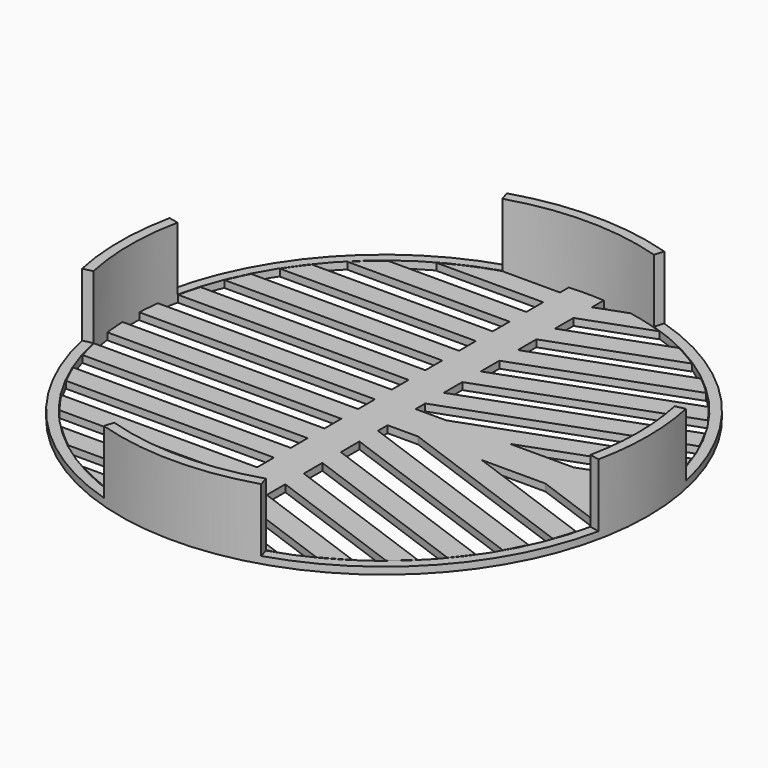
from build123d import *

# Parameters (mm, degrees)
F1_R     = 37.5
F1_R_2   = 36.1
F2_DEPTH = 10
F3_R     = 36
F4_DEPTH = 1
F5_DEPTH = 1
F7_DEPTH = 9


with BuildPart() as f2:
    # F1 (on Top) → F2 (new body)
    with BuildSketch(Plane.XY):
        Circle(F1_R)
        Circle(F1_R_2, mode=Mode.SUBTRACT)
    extrude(amount=F2_DEPTH)

    # F6 (on face) → F7 (cut)
    with BuildSketch(Plane.XY.offset(10)):
        with BuildLine():
            Line((-36.7841187228, 7.7902894544), (-35.316667178, 7.4795066305))
            ThreePointArc((-35.316667178, 7.4795066305), (-26.7003142326, 24.2961564837), (-10.7688596698, 34.4563733061))
            Line((-10.7688596698, 34.4563733061), (-11.2163192129, 35.8880785682))
            ThreePointArc((-11.2163192129, 35.8880785682), (-27.8097455719, 25.3056920716), (-36.7841187228, 7.7902894544))
        make_face()
        with BuildLine():
            Line((35.316667178, 7.4795066305), (36.7841187228, 7.7902894544))
            ThreePointArc((36.7841187228, 7.7902894544), (27.8097455719, 25.3056920716), (11.2163192129, 35.8880785682))
            Line((11.2163192129, 35.8880785682), (10.7688596698, 34.4563733061))
            ThreePointArc((10.7688596698, 34.4563733061), (26.7003142326, 24.2961564837), (35.316667178, 7.4795066305))
        make_face()
        with BuildLine():
            Line((10.7688596698, -34.4563733061), (11.2163192129, -35.8880785682))
            ThreePointArc((11.2163192129, -35.8880785682), (27.8097455719, -25.3056920716), (36.7841187228, -7.7902894544))
            Line((36.7841187228, -7.7902894544), (35.316667178, -7.4795066305))
            ThreePointArc((35.316667178, -7.4795066305), (26.7003142326, -24.2961564837), (10.7688596698, -34.4563733061))
        make_face()
        with BuildLine():
            Line((-35.316667178, -7.4795066305), (-36.7841187228, -7.7902894544))
            ThreePointArc((-36.7841187228, -7.7902894544), (-27.8097455719, -25.3056920716), (-11.2163192129, -35.8880785682))
            Line((-11.2163192129, -35.8880785682), (-10.7688596698, -34.4563733061))
            ThreePointArc((-10.7688596698, -34.4563733061), (-26.7003142326, -24.2961564837), (-35.316667178, -7.4795066305))
        make_face()
    extrude(amount=-F7_DEPTH, mode=Mode.SUBTRACT)


with BuildPart() as f4:
    # F3 (on Top) → F4 (new body)
    with BuildSketch(Plane.XY):
        Circle(F3_R)
    extrude(amount=F4_DEPTH)

    # F0 (on Top) → F5 (cut)
    with BuildSketch(Plane.XY):
        Polygon((-2.4902910933, -34.3626238759), (-11.0826741202, -34.3626238759), (-10.311164963, -34.6114821287), (-7.0564703338, -35.4167498713), (-3.6922154676, -35.9188919628), (-2.4902910933, -36.009670445), align=None)
        Polygon((7.1067539106, -35.491391156), (2.4903820491, -33.8106669574), (2.4903820491, -36.1048205425), (5.8271119297, -35.7271075774), align=None)
        Polygon((-2.4902910933, -28.3864097812), (-22.3032075436, -28.3864097812), (-21.9489178016, -28.6704298539), (-19.2770242661, -30.5341142514), (-17.8802661697, -31.3744898433), (-2.4902910933, -31.3744898433), align=None)
        Polygon((16.3929284881, -32.2909909103), (2.4903820491, -27.2297667069), (2.4903820491, -30.52097242), (12.2555453479, -34.0756893929), (13.7035754764, -33.5237324744), (15.1834482354, -32.881024059), align=None)
        Polygon((-2.4902910933, -22.4102226717), (-28.2984732461, -22.4102226717), (-27.7919325539, -23.0500436622), (-26.726094947, -24.2767944941), (-25.6602843254, -25.3982757485), (-2.4902910933, -25.3982757485), align=None)
        Polygon((22.877221436, -28.0701422988), (2.4903820491, -20.6488934416), (2.4903820491, -23.9400181989), (19.8775377035, -30.2676885812), (20.7367490209, -29.6967340255), (22.0223277634, -28.7552985597), align=None)
        Polygon((-2.4902910933, -16.4337926948), (-32.1518632989, -16.4337926948), (-31.48424747, -17.687258954), (-30.6497546691, -19.09265234), (-30.4345200753, -19.4221426096), (-2.4902910933, -19.4221426096), align=None)
        Polygon((27.7583188949, -23.2651163443), (2.4903820491, -14.0679931911), (2.4903820491, -17.3591179483), (25.4877774299, -25.7291422675), (25.6105604542, -25.6105419616), (26.7099407642, -24.4612658687), align=None)
        Polygon((-2.4902910933, -10.4576325706), (-34.560191604, -10.4576325706), (-34.1722242324, -11.6843834025), (-33.6012696767, -13.2392752401), (-33.5134056048, -13.4459824855), (-2.4902910933, -13.4459824855), align=None)
        Polygon((31.4199515476, -18.0164793708), (2.4903820491, -7.4870929405), (2.4903820491, -10.7782176978), (29.7260855176, -20.6912603313), (30.5809791902, -19.4073007056), (31.4080780243, -18.0386073005), align=None)
        Polygon((-2.4902910933, -4.4814724464), (-35.8207280066, -4.4814724464), (-35.738773711, -5.1623110626), (-35.4591252536, -6.8340491629), (-35.3229575304, -7.4695525085), (-2.4902910933, -7.4695525085), align=None)
        Polygon((36.1048660204, -2.4902286301), (33.9630443413, -2.4902286301), (36.0374028202, -3.244467208), align=None)
        Polygon((24.9224358124, -2.4902286301), (15.8820971364, -2.4902286301), (34.9512452974, -9.4313823695), (35.0551386257, -9.065192119), (35.4269957851, -7.4592981021), (35.6245280352, -6.3847442497), align=None)
        Polygon((6.8417584603, -2.4902286301), (2.4903820491, -2.4902286301), (2.4903820491, -4.1959681833), (32.8501713912, -15.2467102245), (32.8809346105, -15.1835646691), (33.5237239818, -13.7034220573), (34.0259200439, -12.3843815675), align=None)
        Polygon((-2.4902910933, 1.4949575306), (-36.0696402299, 1.4949575306), (-36.1062052844, -2.69853e-05), (-36.0696402299, -1.4933923843), (-2.4902910933, -1.4933923843), align=None)
        Polygon((36.1048660204, 2.4904445123), (36.0374028202, 3.2454926487), (33.9630443413, 2.4904445123), align=None)
        Polygon((-2.4902910933, 7.4694985379), (-35.3229575304, 7.4694985379), (-35.4591252536, 6.8358841619), (-35.738773711, 5.162257092), (-35.8207280066, 4.4827677399), (-2.4902910933, 4.4827677399), align=None)
        Polygon((35.0551386257, 9.0654080012), (34.9512452974, 9.431328399), (15.8820971364, 2.4904445123), (24.9224358124, 2.4904445123), (35.6245280352, 6.3860395431), (35.4269957851, 7.4595139843), align=None)
        Polygon((-2.4902910933, 13.4456586621), (-33.5134056048, 13.4456586621), (-33.6012696767, 13.2394911224), (-34.1722242324, 11.6845992848), (-34.560191604, 10.4578484528), (-2.4902910933, 10.4578484528), align=None)
        Polygon((32.8809346105, 15.1835106986), (32.8501713912, 15.2466562539), (2.4903820491, 4.1975333295), (2.4903820491, 2.4904445123), (6.8417584603, 2.4904445123), (34.0259200439, 12.384327597), (33.5237239818, 13.7036379396), align=None)
        Polygon((-2.4902910933, 19.4220886391), (-30.4345200753, 19.4220886391), (-30.6497546691, 19.0925983694), (-31.48424747, 17.6872049834), (-32.1518632989, 16.434008577), (-2.4902910933, 16.434008577), align=None)
        Polygon((30.5809791902, 19.4075165879), (29.7260855176, 20.6912063608), (2.4903820491, 10.7781637273), (2.4903820491, 7.48703897), (31.4199515476, 18.0166952531), (31.4080780243, 18.0382834771), align=None)
        Polygon((-2.4902910933, 25.3982487633), (-25.6602843254, 25.3982487633), (-26.726094947, 24.2767405236), (-27.7919325539, 23.0497198388), (-28.2984732461, 22.4098988484), (-2.4902910933, 22.4098988484), align=None)
        Polygon((25.6105604542, 25.6103530646), (25.4877774299, 25.7290882969), (2.4903820491, 17.3593338306), (2.4903820491, 14.0679392205), (27.7583188949, 23.2653322266), (26.7099407642, 24.4626691033), align=None)
        Polygon((20.7367490209, 29.6967340255), (19.8775377035, 30.2690918158), (2.4903820491, 23.9399642283), (2.4903820491, 20.648839471), (22.877221436, 28.0700613429), (22.0223277634, 28.7552176039), align=None)
        Polygon((-2.4902910933, 31.3744088874), (-17.8802661697, 31.3744088874), (-19.2770242661, 30.5340872661), (-21.9489178016, 28.6702139717), (-22.3032075436, 28.3865986782), (-2.4902910933, 28.3865986782), align=None)
        Polygon((13.7035754764, 33.523786445), (12.2555453479, 34.0756354224), (2.4903820491, 30.5208644788), (2.4903820491, 27.2313588384), (16.3929284881, 32.2910988514), (15.1834482354, 32.8809970737), align=None)
        Polygon((-2.4902910933, 34.3624889495), (-2.4902910933, 36.011019709), (-3.6922154676, 35.9187300511), (-7.0564703338, 35.416533989), (-10.311164963, 34.6115630846), (-11.0826741202, 34.3624889495), align=None)
        Polygon((5.8271119297, 35.7271345626), (2.4903820491, 36.1062777476), (2.4903820491, 33.8119892361), (7.1067539106, 35.4915530676), align=None)
    extrude(amount=F5_DEPTH, mode=Mode.SUBTRACT)


solid = Compound([f2.part, f4.part])
